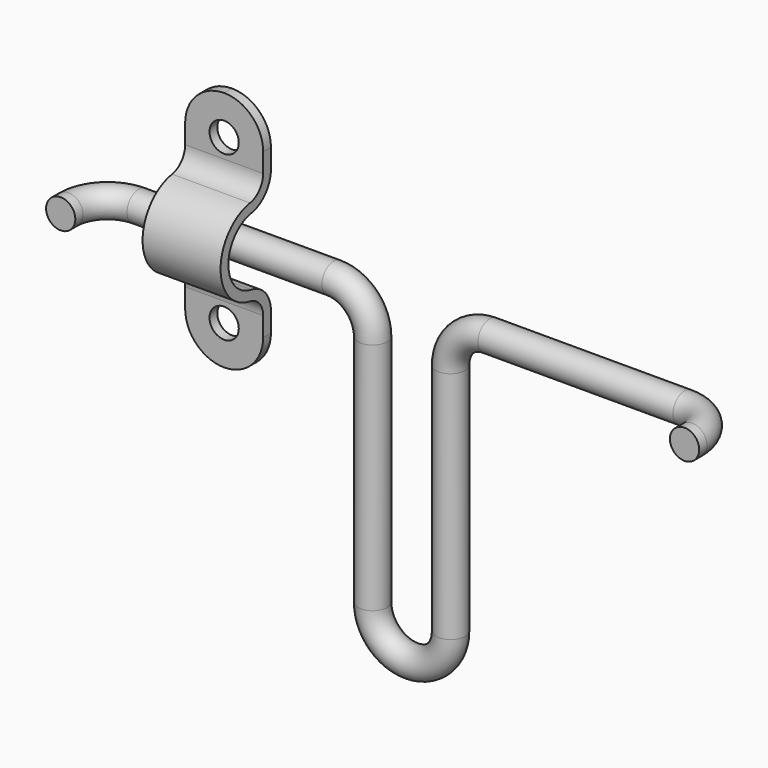
from build123d import *

# Parameters (mm, degrees)
F2_R      = 4.7625
F5_ANGLE  = 90
F6_DEPTH  = 3.175
F11_DEPTH = 25.4
F12_R     = 12.69999
F13_R     = 4.7625
F14_DEPTH = 3.176


# Not quite as in the source:
# - a fillet or chamfer is up to 0.001 mm smaller than in the source, because OpenCascade refuses the exact size
# - a feature names something its author has since deleted; it is built from what else it names


with BuildPart() as f3:
    # F3: sweep along a path in F0
    with BuildLine(Plane.XZ) as f3_path:
        Line((88.9, 88.9), (25.4, 88.9))
        ThreePointArc((25.4, 88.9), (16.4197438789, 85.1802561211), (12.7, 76.2))
        Line((12.7, 76.2), (12.7, 0))
        ThreePointArc((12.7, 0), (0, -12.7), (-12.7, 0))
        Line((-12.7, 0), (-12.7, 76.2))
        ThreePointArc((-12.7, 76.2), (-16.4197438789, 85.1802561211), (-25.4, 88.9))
        Line((-25.4, 88.9), (-88.9, 88.9))
    # F2 (on line) → F3 (sweep)
    with BuildSketch(Plane.YZ.offset(88.9)):
        with Locations((0, 88.9)):
            Circle(F2_R)
    sweep(path=f3_path.line)

    # F2 (on line) → F5 (revolve)
    with BuildSketch(Plane.YZ.offset(88.9)):
        with Locations((0, 88.9)):
            Circle(F2_R)
    revolve(axis=Axis((88.9, -12.7, 113.1016425788), (0, 0, -1)), revolution_arc=F5_ANGLE)

    # F6 (add): a face of the model
    f6_faces = [f3.faces().sort_by_distance(p)[0] for p in [
        (101.6, -12.7, 88.9),
    ]]
    extrude(f6_faces, amount=F6_DEPTH)


with BuildPart() as f7_1:
    # F7: instance of F3
    add(f3.part.mirror(Plane.YZ))

    # F8: union F3
    add(f3.part)


with BuildPart() as f11:
    # F10 (on offset) → F11 (new body)
    with BuildSketch(Plane.YZ.offset(-76.2)):
        with BuildLine():
            ThreePointArc((3.048, 109.2716273834), (1.5340159222, 105.15635704), (-2.286, 103.0034343424))
            ThreePointArc((-2.286, 103.0034343424), (-14.2875, 88.9), (-2.286, 74.7965656576))
            ThreePointArc((-2.286, 74.7965656576), (1.5340159222, 72.64364296), (3.048, 68.5283726166))
            Line((3.048, 68.5283726166), (3.048, 49.5414057925))
            Line((3.048, 49.5414057925), (6.223, 49.5414057925))
            Line((6.223, 49.5414057925), (6.223, 68.5283726166))
            ThreePointArc((6.223, 68.5283726166), (3.9520238833, 74.7012781318), (-1.778, 77.9306621781))
            ThreePointArc((-1.778, 77.9306621781), (-11.1125, 88.9), (-1.778, 99.8693378219))
            ThreePointArc((-1.778, 99.8693378219), (3.9520238833, 103.0987218682), (6.223, 109.2716273834))
            Line((6.223, 109.2716273834), (6.223, 128.2585942075))
            Line((6.223, 128.2585942075), (3.048, 128.2585942075))
            Line((3.048, 128.2585942075), (3.048, 109.2716273834))
        make_face()
    extrude(amount=F11_DEPTH)

    # F12 (radius 12.7 in the source; OpenCascade refuses exactly that, so slightly less here)
    f12_edges = [f11.edges().sort_by_distance(p)[0] for p in [
        (-76.2, 4.6355, 128.258594),
        (-50.8, 4.6355, 128.258594),
        (-50.8, 4.6355, 49.541406),
        (-76.2, 4.6355, 49.541406),
    ]]
    fillet(f12_edges, radius=F12_R)

    # F13 (on face) → F14 (cut, through all)
    with BuildSketch(Plane.XZ.offset(-3.048)):
        with Locations((-63.5, 115.5585942075)):
            Circle(F13_R)
        with Locations((-63.5, 62.2414057925)):
            Circle(F13_R)
    extrude(amount=-F14_DEPTH, mode=Mode.SUBTRACT)


solid = Compound([f7_1.part, f11.part])
